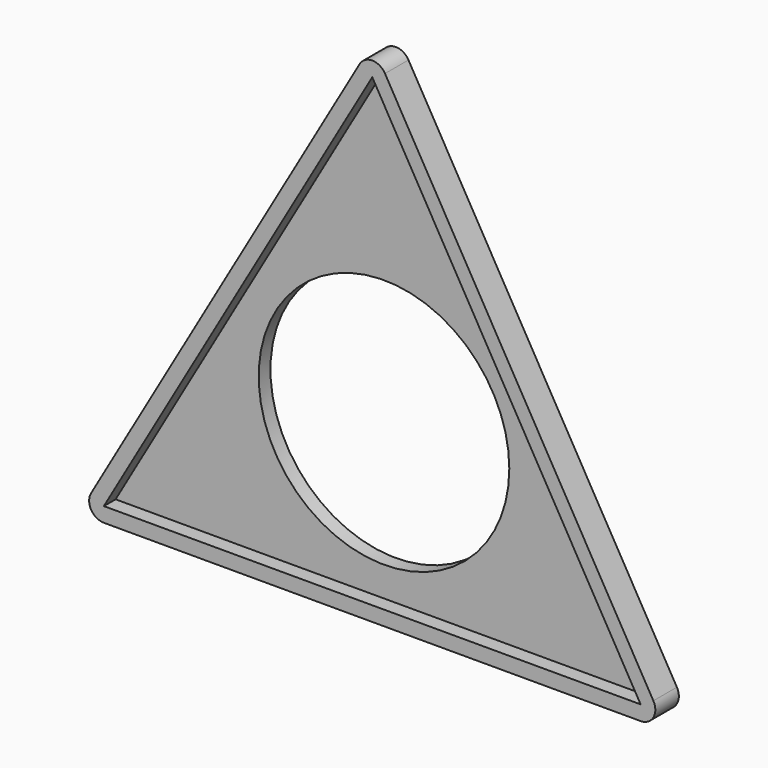
from build123d import *

# Parameters (mm, degrees)
F1_DEPTH = 2.54
F2_R     = 1.27
F3_T     = 1.27
F4_R     = 10.8314490516
F5_DEPTH = 1.271


# Not quite as in the source:
# - a shell that OpenCascade refuses in one call is made with other operations: the cavity is built on its own and cut out


with BuildPart() as f1:
    # F0 (on Front) → F1 (new body)
    with BuildSketch(Plane.XZ):
        Polygon((25.4, -14.6646968374), (0, 29.3293936748), (-25.4, -14.6646968374), align=None)
    extrude(amount=F1_DEPTH)

    # F2
    f2_edges = [f1.edges().sort_by_distance(p)[0] for p in [
        (-25.4, -1.27, -14.664697),
        (25.4, -1.27, -14.664697),
        (0, -1.27, 29.329394),
    ]]
    fillet(f2_edges, radius=F2_R)

    # F3: shell of thickness 1.27, made by hand


with BuildPart() as f3_core1:
    # F3_t2: copy of F1
    add(f1.part)

    # the walls: a layer under each face that stays
    f3_faces = [f3_core1.faces().sort_by_distance(p)[0] for p in [
        (12.7, -1.27, 7.3323484187),
        (0, 0, 6.6973484187),
        (0, -1.27, -14.6646968374),
        (-12.7, -1.27, 7.3323484187),
    ]]
    thicken(f3_faces, amount=-F3_T, mode=Mode.SUBTRACT)


with BuildPart() as f1_1:
    add(f1.part)

    # what is left inside the walls is the cavity
    f3_cavity = [f3_core1.part.solids().sort_by_distance(p)[0] for p in [
        (0, -1.2827, 0),
    ]]
    add(f3_cavity, mode=Mode.SUBTRACT)

    # F4 (on face) → F5 (cut, through all)
    with BuildSketch(Plane.XZ.offset(1.27)):
        Circle(F4_R)
    extrude(amount=-F5_DEPTH, mode=Mode.SUBTRACT)


solid = f1_1.part
